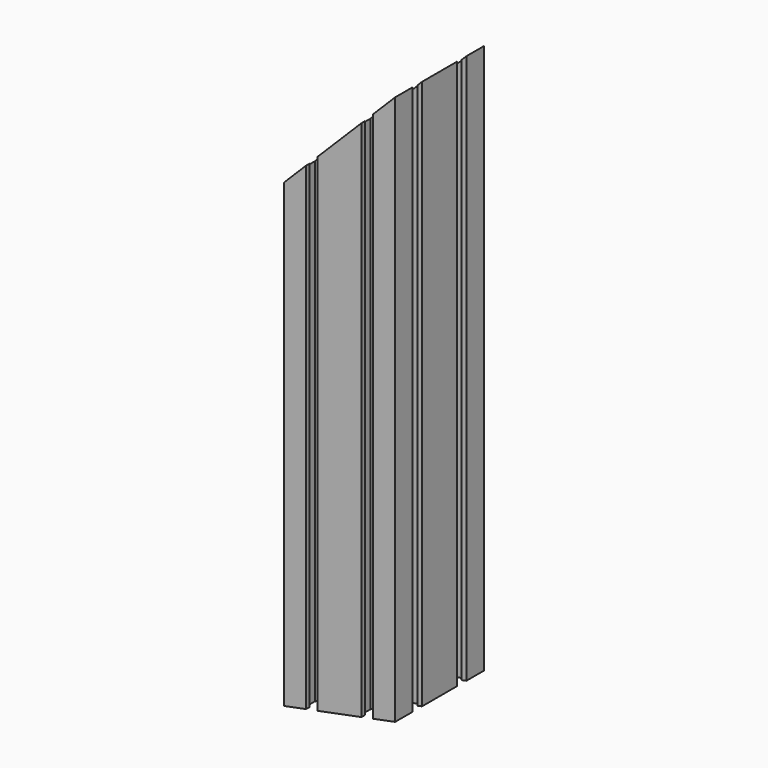
from build123d import *

# Parameters (mm, degrees)
F0_R          = 3
F0_R_2        = 2.5
F1_DEPTH      = 309.2
F2_R          = 2
F3_R          = 7
F6_DEPTH      = 30
F6_DEPTH_BACK = 30


# Not quite as in the source:
# - a feature names something its author has since deleted; it is built from what else it names


with BuildPart() as f1:
    # F0 (on Top) → F1 (new body)
    with BuildSketch(Plane.XY):
        with BuildLine():
            Line((18.15, -30), (30, -30))
            Line((30, -30), (30, -18.15))
            Line((30, -18.15), (27.5, -18.15))
            Line((27.5, -18.15), (27.5, -20.15))
            Line((27.5, -20.15), (21.5477069044, -20.15))
            ThreePointArc((21.5477069044, -20.15), (19.5, -15), (21.5477069044, -9.85))
            Line((21.5477069044, -9.85), (27.5, -9.85))
            Line((27.5, -9.85), (27.5, -11.85))
            Line((27.5, -11.85), (30, -11.85))
            Line((30, -11.85), (30, 11.85))
            Line((30, 11.85), (27.5, 11.85))
            Line((27.5, 11.85), (27.5, 9.85))
            Line((27.5, 9.85), (21.5477069044, 9.85))
            ThreePointArc((21.5477069044, 9.85), (19.5, 15), (21.5477069044, 20.15))
            Line((21.5477069044, 20.15), (27.5, 20.15))
            Line((27.5, 20.15), (27.5, 18.15))
            Line((27.5, 18.15), (30, 18.15))
            Line((30, 18.15), (30, 30))
            Line((30, 30), (18.15, 30))
            Line((18.15, 30), (18.15, 27.5))
            Line((18.15, 27.5), (20.15, 27.5))
            Line((20.15, 27.5), (20.15, 21.5477069044))
            ThreePointArc((20.15, 21.5477069044), (15, 19.5), (9.85, 21.5477069044))
            Line((9.85, 21.5477069044), (9.85, 27.5))
            Line((9.85, 27.5), (11.85, 27.5))
            Line((11.85, 27.5), (11.85, 30))
            Line((11.85, 30), (-11.85, 30))
            Line((-11.85, 30), (-11.85, 27.5))
            Line((-11.85, 27.5), (-9.85, 27.5))
            Line((-9.85, 27.5), (-9.85, 21.5477069044))
            ThreePointArc((-9.85, 21.5477069044), (-15, 19.5), (-20.15, 21.5477069044))
            Line((-20.15, 21.5477069044), (-20.15, 27.5))
            Line((-20.15, 27.5), (-18.15, 27.5))
            Line((-18.15, 27.5), (-18.15, 30))
            Line((-18.15, 30), (-30, 30))
            Line((-30, 30), (-30, 18.15))
            Line((-30, 18.15), (-27.5, 18.15))
            Line((-27.5, 18.15), (-27.5, 20.15))
            Line((-27.5, 20.15), (-21.5477069044, 20.15))
            ThreePointArc((-21.5477069044, 20.15), (-19.5, 15), (-21.5477069044, 9.85))
            Line((-21.5477069044, 9.85), (-27.5, 9.85))
            Line((-27.5, 9.85), (-27.5, 11.85))
            Line((-27.5, 11.85), (-30, 11.85))
            Line((-30, 11.85), (-30, -11.85))
            Line((-30, -11.85), (-27.5, -11.85))
            Line((-27.5, -11.85), (-27.5, -9.85))
            Line((-27.5, -9.85), (-21.5477069044, -9.85))
            ThreePointArc((-21.5477069044, -9.85), (-19.5, -15), (-21.5477069044, -20.15))
            Line((-21.5477069044, -20.15), (-27.5, -20.15))
            Line((-27.5, -20.15), (-27.5, -18.15))
            Line((-27.5, -18.15), (-30, -18.15))
            Line((-30, -18.15), (-30, -30))
            Line((-30, -30), (-18.15, -30))
            Line((-18.15, -30), (-18.15, -27.5))
            Line((-18.15, -27.5), (-20.15, -27.5))
            Line((-20.15, -27.5), (-20.15, -21.5477069044))
            ThreePointArc((-20.15, -21.5477069044), (-15, -19.5), (-9.85, -21.5477069044))
            Line((-9.85, -21.5477069044), (-9.85, -27.5))
            Line((-9.85, -27.5), (-11.85, -27.5))
            Line((-11.85, -27.5), (-11.85, -30))
            Line((-11.85, -30), (11.85, -30))
            Line((11.85, -30), (11.85, -27.5))
            Line((11.85, -27.5), (9.85, -27.5))
            Line((9.85, -27.5), (9.85, -21.5477069044))
            ThreePointArc((9.85, -21.5477069044), (15, -19.5), (20.15, -21.5477069044))
            Line((20.15, -21.5477069044), (20.15, -27.5))
            Line((20.15, -27.5), (18.15, -27.5))
            Line((18.15, -27.5), (18.15, -30))
        make_face()
        with Locations((-25, -25)):
            Circle(F0_R, mode=Mode.SUBTRACT)
        with Locations((-15, -15)):
            Circle(F0_R_2, mode=Mode.SUBTRACT)
        with Locations((25, -25)):
            Circle(F0_R, mode=Mode.SUBTRACT)
        with Locations((15, -15)):
            Circle(F0_R_2, mode=Mode.SUBTRACT)
        with Locations((-25, 25)):
            Circle(F0_R, mode=Mode.SUBTRACT)
        with Locations((-15, 15)):
            Circle(F0_R_2, mode=Mode.SUBTRACT)
        Polygon((-7, 22), (-7, 27.5), (0, 27.5), (7, 27.5), (7, 22), (10, 16), (10, 10), (16, 10), (22, 7), (27.5, 7), (27.5, 0), (27.5, -7), (22, -7), (16, -10), (10, -10), (10, -16), (7, -22), (7, -27.5), (0, -27.5), (-7, -27.5), (-7, -22), (-10, -16), (-10, -10), (-16, -10), (-22, -7), (-27.5, -7), (-27.5, 0), (-27.5, 7), (-22, 7), (-16, 10), (-10, 10), (-10, 16), align=None, mode=Mode.SUBTRACT)
        with Locations((15, 15)):
            Circle(F0_R_2, mode=Mode.SUBTRACT)
        with Locations((25, 25)):
            Circle(F0_R, mode=Mode.SUBTRACT)
    extrude(amount=F1_DEPTH)

    # F2
    f2_edges = [f1.edges().sort_by_distance(p)[0] for p in [
        (-7, 27.5, 154.6),
        (7, 27.5, 154.6),
    ]]
    fillet(f2_edges, radius=F2_R)

    # F3
    f3_edges = [f1.edges().sort_by_distance(p)[0] for p in [
        (-10, 16, 154.6),
        (10, 16, 154.6),
    ]]
    fillet(f3_edges, radius=F3_R)

    # F5 (on Front) → F6 (cut, two sides)
    with BuildSketch(Plane.XZ) as f6_sk:
        Polygon((199.6708250374, -78.6542790774), (175.8796550084, 40.952009573), (-30, 0), (-6.208829971, -119.6062886505), align=None)
        Polygon((30, 309.2), (-52.0743704197, 391.2743704197), (-206.6919281066, 236.6568127329), (-124.6175576868, 154.5824423132), align=None)
    extrude(amount=F6_DEPTH, mode=Mode.SUBTRACT)
    extrude(f6_sk.sketch, amount=-F6_DEPTH_BACK, mode=Mode.SUBTRACT)


solid = f1.part
